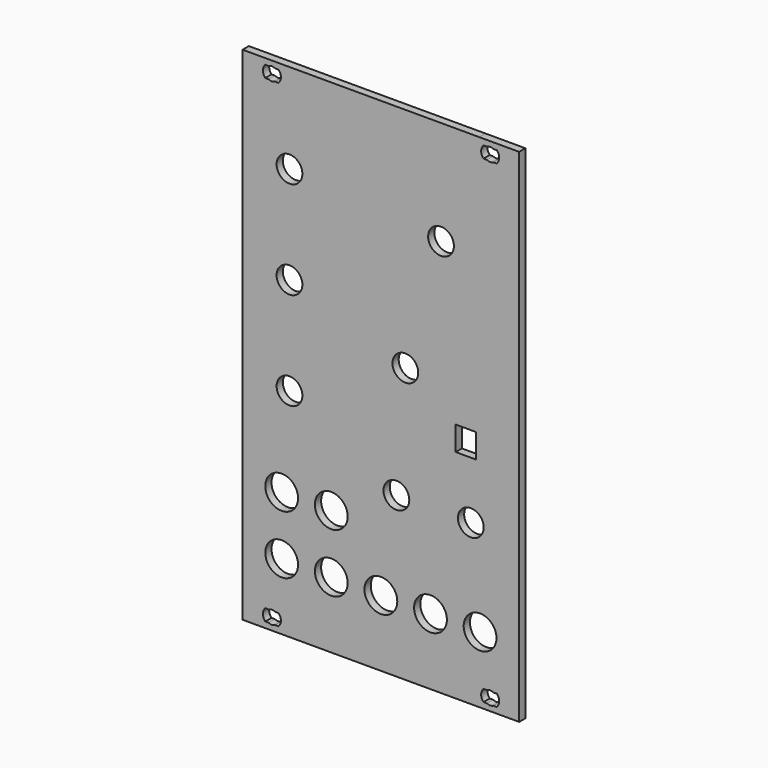
from build123d import *

# Parameters (mm, degrees)
F0_R     = 4.199999
F0_R_2   = 3.300001
F0_W     = 5.2
F0_H     = 6.199998
F1_DEPTH = 2


# Not quite as in the source:
# - ends of sketch curves that miss each other by under 0.0002 mm in the source are joined


with BuildPart() as f1:
    # F0 (on Front) → F1 (new body)
    with BuildSketch(Plane.XZ):
        Polygon((-35.399994, -61.250012), (-35.399994, -64.250012), (35.399993, -64.250012), (35.399993, 64.250001), (25.199994, 64.250011), (15.100006, 64.250011), (-35.399994, 64.250011), align=None)
        with BuildLine():
            Line((-28.699995, -62.750012), (-29.599993, -62.750012))
            ThreePointArc((-29.599993, -62.750012), (-30.199994, -61.2500123621), (-29.5999938002, -59.7500141903))
            Line((-29.5999938002, -59.7500141903), (-28.699995, -59.750013))
            ThreePointArc((-28.699995, -59.750013), (-27.8999944412, -59.550011), (-27.099993, -59.750013))
            Line((-27.099993, -59.750013), (-26.199995, -59.750013))
            ThreePointArc((-26.199995, -59.750013), (-25.599994, -61.2500123621), (-26.1999951748, -62.7500108335))
            Line((-26.1999951748, -62.7500108335), (-27.099993, -62.750012))
            ThreePointArc((-27.099993, -62.750012), (-27.8999944412, -62.950014), (-28.699995, -62.750012))
        make_face(mode=Mode.SUBTRACT)
        with Locations((-25.400037, -47.249964)):
            Circle(F0_R, mode=Mode.SUBTRACT)
        with Locations((-25.400037, -32.249966)):
            Circle(F0_R, mode=Mode.SUBTRACT)
        with Locations((-12.700012, -47.249939)):
            Circle(F0_R, mode=Mode.SUBTRACT)
        with Locations((-12.700063, -32.249938)):
            Circle(F0_R, mode=Mode.SUBTRACT)
        with Locations((-3.7e-05, -47.249964)):
            Circle(F0_R, mode=Mode.SUBTRACT)
        with Locations((-23.400008, -8.750001)):
            Circle(F0_R_2, mode=Mode.SUBTRACT)
        with Locations((12.699963, -47.249964)):
            Circle(F0_R, mode=Mode.SUBTRACT)
        with BuildLine():
            ThreePointArc((27.179992, -59.75), (27.9799934412, -59.549998), (28.7799947785, -59.7500004152))
            Line((28.7799947785, -59.7500004152), (29.679992, -59.75))
            ThreePointArc((29.679992, -59.75), (30.279993, -61.25), (29.6799923008, -62.7499983341))
            Line((29.6799923008, -62.7499983341), (28.779994, -62.749999))
            ThreePointArc((28.779994, -62.749999), (27.9799934412, -62.950001), (27.179992, -62.749999))
            Line((27.179992, -62.749999), (26.279994, -62.749999))
            ThreePointArc((26.279994, -62.749999), (25.679993, -61.25), (26.2799941748, -59.7500011665))
            Line((26.2799941748, -59.7500011665), (27.179992, -59.75))
        make_face(mode=Mode.SUBTRACT)
        with Locations((25.400013, -47.249921)):
            Circle(F0_R, mode=Mode.SUBTRACT)
        with Locations((3.969993, -23.379999)):
            Circle(F0_R_2, mode=Mode.SUBTRACT)
        with Locations((23.019993, -23.379999)):
            Circle(F0_R_2, mode=Mode.SUBTRACT)
        with Locations((21.74983, -5.600162)):
            Rectangle(F0_W, F0_H, mode=Mode.SUBTRACT)
        with Locations((-23.400008, 16.25)):
            Circle(F0_R_2, mode=Mode.SUBTRACT)
        with Locations((-23.400008, 41.250001)):
            Circle(F0_R_2, mode=Mode.SUBTRACT)
        with BuildLine():
            Line((-28.700008, 59.750002), (-29.600006, 59.750002))
            ThreePointArc((-29.600006, 59.750002), (-30.200007, 61.250002), (-29.6000038751, 62.7500028811))
            Line((-29.6000038751, 62.7500028811), (-28.700008, 62.750001))
            ThreePointArc((-28.700008, 62.750001), (-27.9000065588, 62.950003), (-27.1000052215, 62.7500005848))
            Line((-27.1000052215, 62.7500005848), (-26.200008, 62.750001))
            ThreePointArc((-26.200008, 62.750001), (-25.600007, 61.250002), (-26.2000076992, 59.7500036659))
            Line((-26.2000076992, 59.7500036659), (-27.100006, 59.750002))
            ThreePointArc((-27.100006, 59.750002), (-27.9000065588, 59.55), (-28.700008, 59.750002))
        make_face(mode=Mode.SUBTRACT)
        with Locations((6.268744, 6.048941)):
            Circle(F0_R_2, mode=Mode.SUBTRACT)
        with Locations((15.399993, 37.580001)):
            Circle(F0_R_2, mode=Mode.SUBTRACT)
        with BuildLine():
            Line((27.179992, 59.750025), (26.279994, 59.750025))
            ThreePointArc((26.279994, 59.750025), (25.679993, 61.2500246379), (26.2799936754, 62.7500233092))
            Line((26.2799936754, 62.7500233092), (27.179992, 62.750024))
            ThreePointArc((27.179992, 62.750024), (27.9799934412, 62.950026), (28.7799947785, 62.7500235848))
            Line((28.7799947785, 62.7500235848), (29.679992, 62.750024))
            ThreePointArc((29.679992, 62.750024), (30.279993, 61.2500246379), (29.6799923008, 59.7500266659))
            Line((29.6799923008, 59.7500266659), (28.779994, 59.750025))
            ThreePointArc((28.779994, 59.750025), (27.9799934412, 59.550023), (27.179992, 59.750025))
        make_face(mode=Mode.SUBTRACT)
    extrude(amount=F1_DEPTH)


solid = f1.part
